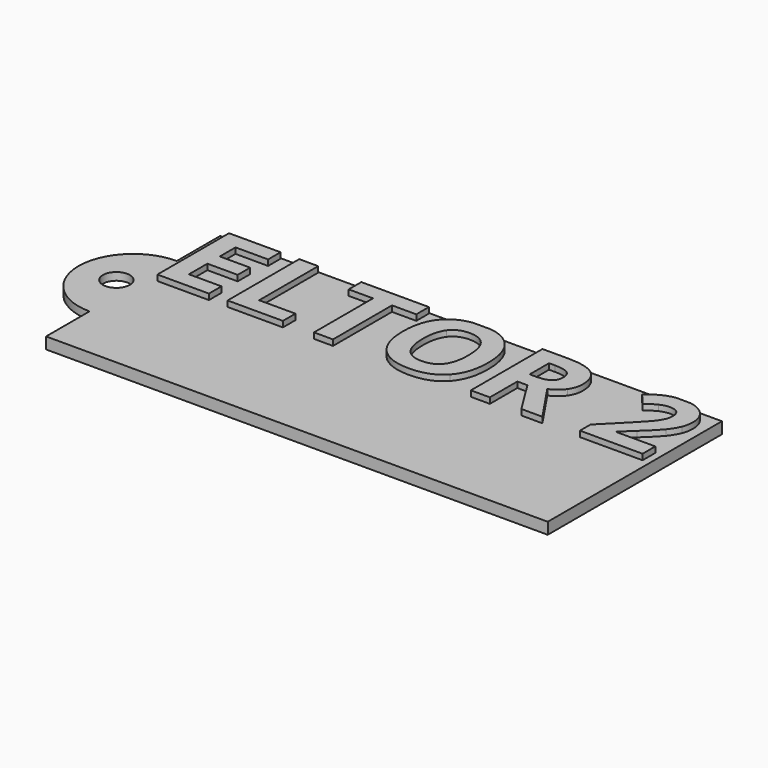
from build123d import *

# Parameters (mm, degrees)
F0_W     = 130.8541893959
F0_H     = 56.7789375782
F1_DEPTH = 3
F3_DEPTH = 1.5
F4_R     = 14.2398683788
F5_DEPTH = 2
F7_D     = 7


# Not quite as in the source:
# - a feature names something its author has since deleted; it is built from what else it names


with BuildPart() as f1:
    # F0 (on Top) → F1 (new body)
    with BuildSketch(Plane.XY):
        Rectangle(F0_W, F0_H)
    extrude(amount=F1_DEPTH)

    # F2 (on face) → F3 (join)
    with BuildSketch(Plane.XY.offset(3)):
        with BuildLine():
            Line((57.2191747598, 28.3894687891), (53.5310418569, 28.3894687891))
            add(Edge.make_bspline(
                [(52.5161502643, 28.1952754595), (53.0025964919, 28.3138756826), (53.5310418569, 28.3894687891)],
                knots=[0, 0, 0, 0.3626225608, 0.3626225608, 0.3626225608], degree=2))
            add(Edge.make_bspline(
                [(50.0401853118, 27.2626364423), (51.1746831848, 27.8682130096), (52.5161502643, 28.1952754595)],
                knots=[0, 0, 0, 1, 1, 1], degree=2))
            add(Edge.make_bspline(
                [(47.1834992262, 25.1852788506), (48.9056874388, 26.657059875), (50.0401853118, 27.2626364423)],
                knots=[0, 0, 0, 1, 1, 1], degree=2))
            Line((47.1834992262, 25.1852788506), (49.8664333853, 22.0066406659))
            add(Edge.make_bspline(
                [(52.534036492, 23.7799323863), (51.2564487973, 23.1564695912), (49.8664333853, 22.0066406659)],
                knots=[0, 0, 0, 1, 1, 1], degree=2))
            add(Edge.make_bspline(
                [(55.1658671433, 24.4033951813), (53.8116241868, 24.4033951813), (52.534036492, 23.7799323863)],
                knots=[0, 0, 0, 1, 1, 1], degree=2))
            add(Edge.make_bspline(
                [(57.2355592089, 23.7160530015), (56.4587858905, 24.4033951813), (55.1658671433, 24.4033951813)],
                knots=[0, 0, 0, 1, 1, 1], degree=2))
            add(Edge.make_bspline(
                [(58.0123325273, 21.6233643575), (58.0123325273, 23.0287108217), (57.2355592089, 23.7160530015)],
                knots=[0, 0, 0, 1, 1, 1], degree=2))
            add(Edge.make_bspline(
                [(57.6597183236, 19.8040794801), (58.0123325273, 20.6830598141), (58.0123325273, 21.6233643575)],
                knots=[0, 0, 0, 1, 1, 1], degree=2))
            add(Edge.make_bspline(
                [(56.5098893983, 17.8953634641), (57.3071041198, 18.9250991461), (57.6597183236, 19.8040794801)],
                knots=[0, 0, 0, 1, 1, 1], degree=2))
            add(Edge.make_bspline(
                [(53.1063957793, 14.1980246753), (55.7126746767, 16.865627782), (56.5098893983, 17.8953634641)],
                knots=[0, 0, 0, 1, 1, 1], degree=2))
            Line((53.1063957793, 14.1980246753), (47.2448234356, 8.2751281222))
            Line((47.2448234356, 8.2751281222), (47.2448234356, 4.8409723986))
            Line((47.2448234356, 4.8409723986), (63.5672838243, 4.8409723986))
            Line((63.5672838243, 4.8409723986), (63.5672838243, 8.9956875821))
            Line((63.5672838243, 8.9956875821), (53.3925754229, 8.9956875821))
            Line((53.3925754229, 8.9956875821), (53.3925754229, 9.2154326656))
            Line((53.3925754229, 9.2154326656), (56.3974616811, 12.0414566465))
            add(Edge.make_bspline(
                [(60.58794932, 16.2753822671), (59.3972375885, 14.7908253657), (56.3974616811, 12.0414566465)],
                knots=[0, 0, 0, 1, 1, 1], degree=2))
            add(Edge.make_bspline(
                [(62.3459099881, 19.1729511588), (61.7786610516, 17.7599391684), (60.58794932, 16.2753822671)],
                knots=[0, 0, 0, 1, 1, 1], degree=2))
            add(Edge.make_bspline(
                [(62.9131589246, 22.2008339955), (62.9131589246, 20.5859631493), (62.3459099881, 19.1729511588)],
                knots=[0, 0, 0, 1, 1, 1], degree=2))
            add(Edge.make_bspline(
                [(61.9856302581, 25.4893447219), (62.9131589246, 24.0507809776), (62.9131589246, 22.2008339955)],
                knots=[0, 0, 0, 1, 1, 1], degree=2))
            add(Edge.make_bspline(
                [(59.3819065362, 27.7251231878), (61.0581015917, 26.9279084663), (61.9856302581, 25.4893447219)],
                knots=[0, 0, 0, 1, 1, 1], degree=2))
            add(Edge.make_bspline(
                [(57.2191747598, 28.3894687891), (58.3900152465, 28.1968763622), (59.3819065362, 27.7251231878)],
                knots=[0.4082482905, 0.4082482905, 0.4082482905, 1, 1, 1], degree=2))
        make_face()
        with BuildLine():
            Line((23.7372098514, 4.8409723986), (23.7372098514, 13.7994173145))
            Line((23.7372098514, 13.7994173145), (26.3690405026, 13.7994173145))
            Line((26.3690405026, 13.7994173145), (31.9444332027, 4.8409723986))
            Line((31.9444332027, 4.8409723986), (37.4380602903, 4.8409723986))
            add(Edge.make_bspline(
                [(30.5697488431, 15.0156808), (35.8436308472, 7.1406302493), (37.4380602903, 4.8409723986)],
                knots=[0, 0, 0, 1, 1, 1], degree=2))
            add(Edge.make_bspline(
                [(33.7816043078, 17.5299733833), (32.6496616103, 15.9253232387), (30.5697488431, 15.0156808)],
                knots=[0, 0, 0, 1, 1, 1], degree=2))
            add(Edge.make_bspline(
                [(34.9135470054, 21.194094892), (34.9135470054, 19.134623528), (33.7816043078, 17.5299733833)],
                knots=[0, 0, 0, 1, 1, 1], degree=2))
            add(Edge.make_bspline(
                [(32.6317753825, 26.4577561946), (34.9135470054, 24.7253472804), (34.9135470054, 21.194094892)],
                knots=[0, 0, 0, 1, 1, 1], degree=2))
            add(Edge.make_bspline(
                [(25.5871568334, 28.1901651087), (30.3500037596, 28.1901651087), (32.6317753825, 26.4577561946)],
                knots=[0, 0, 0, 1, 1, 1], degree=2))
            Line((25.5871568334, 28.1901651087), (18.7852799463, 28.1901651087))
            Line((18.7852799463, 28.1901651087), (18.7852799463, 4.8409723986))
            Line((18.7852799463, 4.8409723986), (23.7372098514, 4.8409723986))
        make_face()
        with BuildLine():
            Line((25.3316392945, 17.8263737285), (23.7372098514, 17.8263737285))
            Line((23.7372098514, 17.8263737285), (23.7372098514, 24.13254659))
            Line((23.7372098514, 24.13254659), (25.2396529804, 24.13254659))
            add(Edge.make_bspline(
                [(28.7734605442, 23.4298733579), (27.6312971451, 24.13254659), (25.2396529804, 24.13254659)],
                knots=[0, 0, 0, 1, 1, 1], degree=2))
            add(Edge.make_bspline(
                [(29.9156239434, 21.0663361225), (29.9156239434, 22.7272001258), (28.7734605442, 23.4298733579)],
                knots=[0, 0, 0, 1, 1, 1], degree=2))
            add(Edge.make_bspline(
                [(28.7990122981, 18.6082573977), (29.9156239434, 19.390141067), (29.9156239434, 21.0663361225)],
                knots=[0, 0, 0, 1, 1, 1], degree=2))
            add(Edge.make_bspline(
                [(25.3316392945, 17.8263737285), (27.6824006529, 17.8263737285), (28.7990122981, 18.6082573977)],
                knots=[0, 0, 0, 1, 1, 1], degree=2))
        make_face(mode=Mode.SUBTRACT)
        with BuildLine():
            add(Edge.make_bspline(
                [(13.9457777584, 16.5487860337), (13.9457777584, 10.7485378994), (11.0712054452, 7.6337790995)],
                knots=[0, 0, 0, 1, 1, 1], degree=2))
            add(Edge.make_bspline(
                [(11.0942020237, 25.4586826172), (13.9457777584, 22.3592548697), (13.9457777584, 16.5487860337)],
                knots=[0, 0, 0, 1, 1, 1], degree=2))
            add(Edge.make_bspline(
                [(5.2342333213, 28.3894687891), (8.9077868298, 27.8351356909), (11.0942020237, 25.4586826172)],
                knots=[0.2332606961, 0.2332606961, 0.2332606961, 1, 1, 1], degree=2))
            Line((5.2342333213, 28.3894687891), (0.4776699233, 28.3894687891))
            add(Edge.make_bspline(
                [(-5.4020102915, 25.4842343711), (-3.1948737915, 27.8381219683), (0.4776699233, 28.3894687891)],
                knots=[0, 0, 0, 0.7657718145, 0.7657718145, 0.7657718145], degree=2))
            add(Edge.make_bspline(
                [(-8.284248131, 16.5794481384), (-8.284248131, 22.4103583775), (-5.4020102915, 25.4842343711)],
                knots=[0, 0, 0, 1, 1, 1], degree=2))
            add(Edge.make_bspline(
                [(-5.4096758177, 7.6337790995), (-8.284248131, 10.7485378994), (-8.284248131, 16.5794481384)],
                knots=[0, 0, 0, 1, 1, 1], degree=2))
            add(Edge.make_bspline(
                [(2.8307648137, 4.5190202995), (-2.5351035044, 4.5190202995), (-5.4096758177, 7.6337790995)],
                knots=[0, 0, 0, 1, 1, 1], degree=2))
            add(Edge.make_bspline(
                [(11.0712054452, 7.6337790995), (8.1966331319, 4.5190202995), (2.8307648137, 4.5190202995)],
                knots=[0, 0, 0, 1, 1, 1], degree=2))
        make_face()
        with BuildLine():
            add(Edge.make_bspline(
                [(-3.0921317393, 16.5487860337), (-3.0921317393, 12.6342573369), (-1.607574838, 10.65399641)],
                knots=[0, 0, 0, 1, 1, 1], degree=2))
            add(Edge.make_bspline(
                [(-1.5922437857, 22.4461308329), (-3.0921317393, 20.4582043798), (-3.0921317393, 16.5487860337)],
                knots=[0, 0, 0, 1, 1, 1], degree=2))
            add(Edge.make_bspline(
                [(2.8614269184, 24.434057286), (-0.092355832, 24.434057286), (-1.5922437857, 22.4461308329)],
                knots=[0, 0, 0, 1, 1, 1], degree=2))
            add(Edge.make_bspline(
                [(8.7536613668, 16.5487860337), (8.7536613668, 24.434057286), (2.8614269184, 24.434057286)],
                knots=[0, 0, 0, 1, 1, 1], degree=2))
            add(Edge.make_bspline(
                [(2.8307648137, 8.673735483), (8.7536613668, 8.673735483), (8.7536613668, 16.5487860337)],
                knots=[0, 0, 0, 1, 1, 1], degree=2))
            add(Edge.make_bspline(
                [(-1.607574838, 10.65399641), (-0.1230179366, 8.673735483), (2.8307648137, 8.673735483)],
                knots=[0, 0, 0, 1, 1, 1], degree=2))
        make_face(mode=Mode.SUBTRACT)
        Polygon((-22.1281883918, 4.8409723986), (-17.1762584868, 4.8409723986), (-17.1762584868, 24.0712223807), (-10.8394235206, 24.0712223807), (-10.8394235206, 28.1901651087), (-28.4701337088, 28.1901651087), (-28.4701337088, 24.0712223807), (-22.1281883918, 24.0712223807), align=None)
        Polygon((-44.664835328, 28.1901651087), (-44.664835328, 4.8409723986), (-30.2434254291, 4.8409723986), (-30.2434254291, 8.929253022), (-39.712905423, 8.929253022), (-39.712905423, 28.1901651087), align=None)
        Polygon((-62.9803325206, 4.8409723986), (-49.5349996205, 4.8409723986), (-49.5349996205, 8.929253022), (-58.0284026155, 8.929253022), (-58.0284026155, 14.9492462399), (-50.1226899601, 14.9492462399), (-50.1226899601, 19.0068647585), (-58.0284026155, 19.0068647585), (-58.0284026155, 24.13254659), (-49.5349996205, 24.13254659), (-49.5349996205, 28.1901651087), (-62.9803325206, 28.1901651087), align=None)
    extrude(amount=F3_DEPTH)

    # F4 (on face) → F5 (join)
    with BuildSketch(Plane.XY.offset(3)):
        with Locations((-65.427094698, 0)):
            Circle(F4_R)
    extrude(amount=-F5_DEPTH)

    # F7 (through all)
    with Locations(Plane.XY.offset(3)):
        with Locations((-69.8119476438, 0)):
            Hole(F7_D / 2)


solid = f1.part
